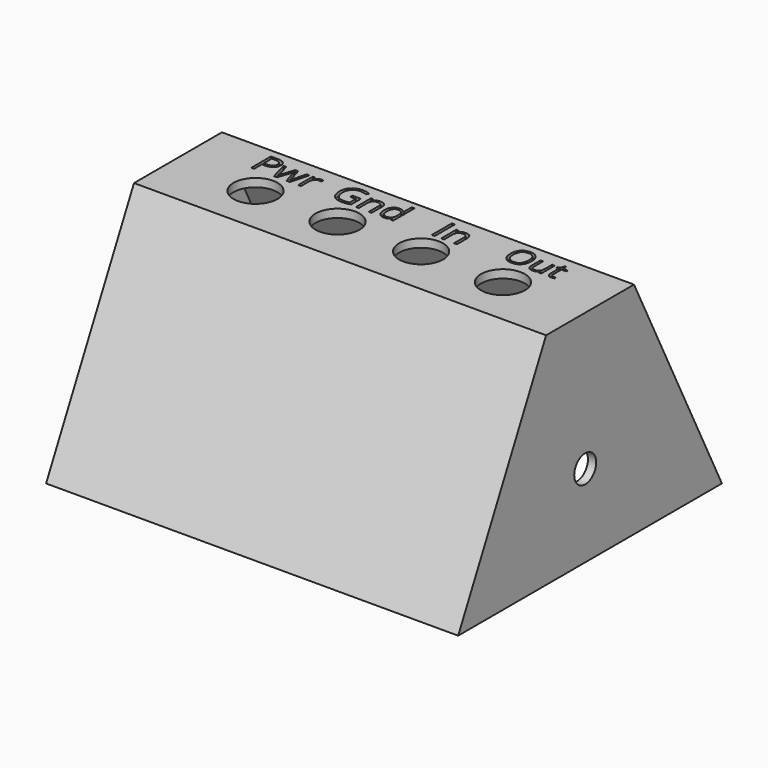
from build123d import *

# Parameters (mm, degrees)
F1_DEPTH       = 75
F2_T           = -1.5
F5_D           = 5
F5_DEPTH       = 20
F5_TIP         = 1.5021515476
F6_TEXT_SIZE   = 5.7981500416
F6_TEXT_SIZE_2 = 6.4131047873
F6_TEXT_SIZE_3 = 6.4131053576
F6_TEXT_SIZE_4 = 6.2374035129
F7_DEPTH       = 0.75
F8_D           = 8


# Not quite as in the source:
# - Text() gives the source's letters only with a copy of the font that has no kerning and outlines rounded to 1/6400 em; it was checked with that copy


with BuildPart() as f1:
    # F0 (on Right) → F1 (new body)
    with BuildSketch(Plane.YZ):
        Polygon((-8.8991851483, 40), (-28.8991851483, 0), (31.1008148517, 0), (11.1008148517, 40), align=None)
    extrude(amount=F1_DEPTH)

    # F2
    f2_openings = [f1.faces().sort_by_distance(p)[0] for p in [
        (37.5, 1.100815, 0),
    ]]
    offset(amount=F2_T, openings=f2_openings)

    # F5
    with Locations(Plane.YZ.offset(75)):
        with Locations((0, 15)):
            Hole(F5_D / 2, depth=F5_DEPTH)
            with Locations((0, 0, -(F5_DEPTH + F5_TIP / 2))):  # 118° drill point
                Cone(0, F5_D / 2, F5_TIP, mode=Mode.SUBTRACT)

    # F6 (on face) → F7 (cut)
    with BuildSketch(Plane.XY.offset(40)):
        with Locations((55.0004545306, 5.5015479881)):
            Text('Out', F6_TEXT_SIZE, font='Open Sans', text_align=(TextAlign.LEFT, TextAlign.BOTTOM))
        with Locations((42.3961792516, 5.0587805712)):
            Text('In', F6_TEXT_SIZE_2, font='Open Sans', text_align=(TextAlign.LEFT, TextAlign.BOTTOM))
        with Locations((24.0082557053, 5.0587801606)):
            Text('Gnd', F6_TEXT_SIZE_3, font='Open Sans', text_align=(TextAlign.LEFT, TextAlign.BOTTOM))
        with Locations((9.4677154624, 5.1852854888)):
            Text('Pwr', F6_TEXT_SIZE_4, font='Open Sans', text_align=(TextAlign.LEFT, TextAlign.BOTTOM))
    extrude(amount=-F7_DEPTH, mode=Mode.SUBTRACT)

    # F8 (through all)
    with Locations(Plane.XY.offset(40)):
        with Locations((15, 0), (30, -0.0982353667), (45, 0.1650898642), (60, 0.0323631143)):
            Hole(F8_D / 2)


solid = f1.part
